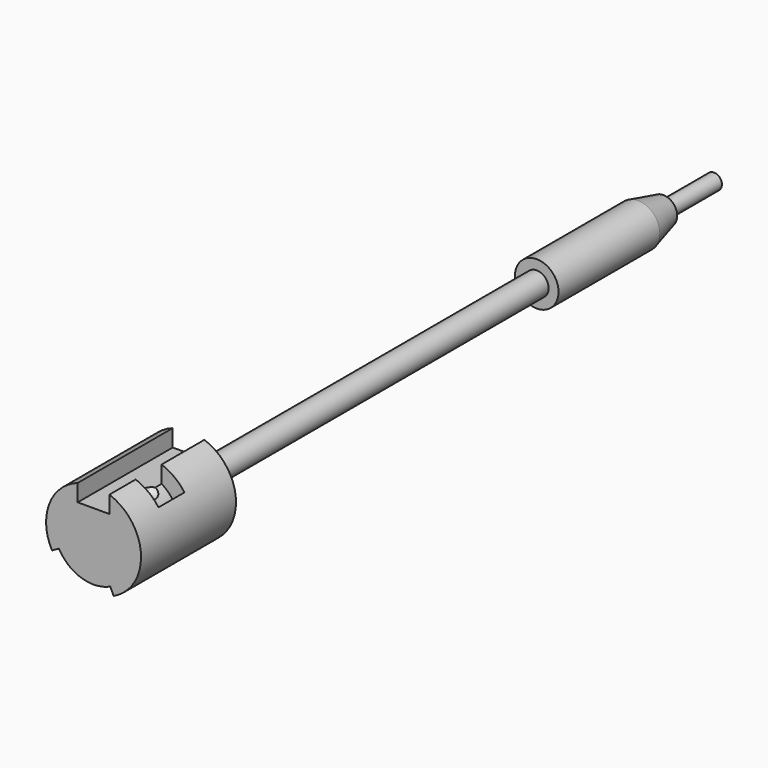
from build123d import *

# Parameters (mm, degrees)
F0_R      = 1
F1_DEPTH  = 8
F2_R      = 2.75
F3_DEPTH  = 80
F4_SIZE2  = 1
F4_SIZE   = 4
F5_R      = 6
F5_R_2    = 2.75
F6_DEPTH  = 5
F7_DEPTH  = 10
F12_R     = 2.75
F12_R_2   = 1.5
F13_DEPTH = 55
F15_D     = 5
F15_DEPTH = 7
F15_START = 0.545644
F15_TIP   = 1.5021515476
F16_W     = 4
F16_H     = 15
F17_DEPTH = 2.5
F19_W     = 4.1
F19_H     = 2.1568542495
F20_ANGLE = 35
F28_DEPTH = 15


with BuildPart() as f1:
    # F0 (on Front) → F1 (new body)
    with BuildSketch(Plane.XZ):
        Circle(F0_R)
    extrude(amount=-F1_DEPTH)

    # F2 (on face) → F3 (join)
    with BuildSketch(Plane.XZ):
        Circle(F2_R)
    extrude(amount=F3_DEPTH)

    # F4
    f4_edges = [f1.edges().sort_by_distance(p)[0] for p in [
        (-2.75, 0, 0),
    ]]
    f4_side = f1.faces().sort_by_distance((-2.75, -40, 0))[0]
    chamfer(f4_edges, length=F4_SIZE, length2=F4_SIZE2, reference=f4_side)

    # F5 (on face) → F6 (join)
    with BuildSketch(Plane.XZ.offset(80)):
        Circle(F5_R)
        Circle(F5_R_2, mode=Mode.SUBTRACT)
    extrude(amount=-F6_DEPTH)

    # F7 (add): a face of the model
    f7_faces = [f1.faces().sort_by_distance(p)[0] for p in [
        (0, -80, 0),
    ]]
    extrude(f7_faces, amount=F7_DEPTH)

    # F12 (on face) → F13 (cut)
    with BuildSketch(Plane(origin=(0, -75, 0), x_dir=(-1, 0, 0), z_dir=(0, 1, 0))):
        Circle(F12_R)
        Circle(F12_R_2, mode=Mode.SUBTRACT)
    extrude(amount=F13_DEPTH, mode=Mode.SUBTRACT)

    # F15
    # its depths count from where the whole tool has entered the part; down to there all is cleared
    with Locations(Plane(origin=(-6, 0, 0), x_dir=(0, 1, 0), z_dir=(-1, 0, 0)).offset(-F15_START)):
        with Locations((-86, 0)):
            Hole(F15_D / 2, depth=F15_DEPTH)
            with Locations((0, 0, -(F15_DEPTH + F15_TIP / 2))):  # 118° drill point
                Cone(0, F15_D / 2, F15_TIP, mode=Mode.SUBTRACT)

    # F16 (on offset) → F17 (cut)
    with BuildSketch(Plane.XY.offset(6)):
        with Locations((0, -82.5)):
            Rectangle(F16_W, F16_H)
    extrude(amount=-F17_DEPTH, mode=Mode.SUBTRACT)

    # F19 (on face) → F20 (revolve, cut)
    with BuildSketch(Plane(origin=(2, 0, 0), x_dir=(0, -1, 0), z_dir=(-1, 0, 0))):
        with Locations((83.8, 4.5784271247)):
            Rectangle(F19_W, F19_H)
    revolve(axis=Axis((0, -80, 0), (0, 1, 0)), revolution_arc=F20_ANGLE, mode=Mode.SUBTRACT)

    # F25 (on face) → F26 (revolve, cut)
    with BuildSketch(Plane(origin=(-0.302441943, 0, 0.2117721284), x_dir=(0, -1, 0), z_dir=(-0.8191520443, 0, 0.5735764364))):
        with BuildLine():
            Line((83.8, 5.9141850277), (83.8, 3.4141850277))
            ThreePointArc((83.8, 3.4141850277), (85.05, 4.6641850277), (83.8, 5.9141850277))
        make_face()
    revolve(axis=Axis((2.3728246836, -83.8, 4.0324488288), (0.5735764364, 0, 0.8191520443)), mode=Mode.SUBTRACT)

    # F27 (on face) → F28 (cut)
    with BuildSketch(Plane.XZ.offset(90)):
        with BuildLine():
            ThreePointArc((-5.2477182428, -2.9088577215), (-1.8541019662, -5.7063390978), (2.5357095704, -5.4378467222))
            Line((2.5357095704, -5.4378467222), (2.1130913087, -4.5315389352))
            ThreePointArc((2.1130913087, -4.5315389352), (-1.5450849719, -4.7552825815), (-4.3730985357, -2.4240481012))
            Line((-4.3730985357, -2.4240481012), (-5.2477182428, -2.9088577215))
        make_face()
    extrude(amount=-F28_DEPTH, mode=Mode.SUBTRACT)


solid = f1.part
